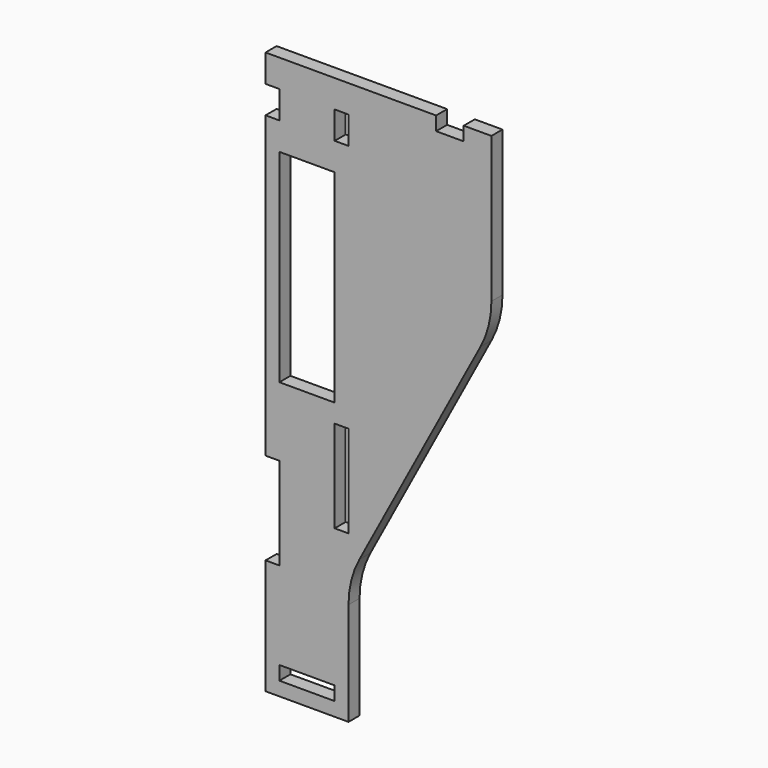
from build123d import *

# Parameters (mm, degrees)
F0_W     = 12
F0_H     = 3
F0_W_2   = 3
F0_H_2   = 20
F0_H_3   = 44
F0_H_4   = 6
F1_DEPTH = 1.5
F3_DEPTH = 1.5


# Not quite as in the source:
# - a feature of the source that left no trace in its solid (it failed there, or was rolled back) is left out


with BuildPart() as f1:
    # F0 (on Front) → F1 (new body, symmetric)
    with BuildSketch(Plane.XZ):
        with BuildLine():
            Line((-147.1994572369, 90.198807884), (-184.1994572369, 90.198807884))
            Line((-184.1994572369, 90.198807884), (-184.1994572369, 84.198807884))
            Line((-184.1994572369, 84.198807884), (-181.1994572369, 84.198807884))
            Line((-181.1994572369, 84.198807884), (-181.1994572369, 78.198807884))
            Line((-181.1994572369, 78.198807884), (-184.1994572369, 78.198807884))
            Line((-184.1994572369, 78.198807884), (-184.1994572369, 13.198807884))
            Line((-184.1994572369, 13.198807884), (-181.1994572369, 13.198807884))
            Line((-181.1994572369, 13.198807884), (-181.1994572369, -6.801192116))
            Line((-181.1994572369, -6.801192116), (-184.1994572369, -6.801192116))
            Line((-184.1994572369, -6.801192116), (-184.1994572369, -31.801192116))
            Line((-184.1994572369, -31.801192116), (-166.1994572369, -31.801192116))
            Line((-166.1994572369, -31.801192116), (-166.1994572369, -9.4251137796))
            ThreePointArc((-166.1994572369, -9.4251137796), (-165.6004708263, -4.5670615257), (-163.8393900667, 0))
            Line((-163.8393900667, 0), (-137.559524407, 49.1850895229))
            ThreePointArc((-137.559524407, 49.1850895229), (-135.7984436474, 53.7521510486), (-135.1994572369, 58.6102033025))
            Line((-135.1994572369, 58.6102033025), (-135.1994572369, 90.198807884))
            Line((-135.1994572369, 90.198807884), (-141.1994572369, 90.198807884))
            Line((-141.1994572369, 90.198807884), (-141.1994572369, 87.198807884))
            Line((-141.1994572369, 87.198807884), (-147.1994572369, 87.198807884))
            Line((-147.1994572369, 87.198807884), (-147.1994572369, 90.198807884))
        make_face()
        with Locations((-175.1994572369, -27.301192116)):
            Rectangle(F0_W, F0_H, mode=Mode.SUBTRACT)
        with Locations((-167.6994572369, 14.198807884)):
            Rectangle(F0_W_2, F0_H_2, mode=Mode.SUBTRACT)
        with Locations((-175.1994572369, 50.198807884)):
            Rectangle(F0_W, F0_H_3, mode=Mode.SUBTRACT)
        with Locations((-167.6994572369, 81.198807884)):
            Rectangle(F0_W_2, F0_H_4, mode=Mode.SUBTRACT)
    extrude(amount=F1_DEPTH, both=True)

    # F0 (on Front) → F3 (cut, symmetric)
    with BuildSketch(Plane.XZ):
        with Locations((-175.1994572369, -27.301192116)):
            Rectangle(F0_W, F0_H)
    extrude(amount=F3_DEPTH, both=True, mode=Mode.SUBTRACT)


solid = f1.part
